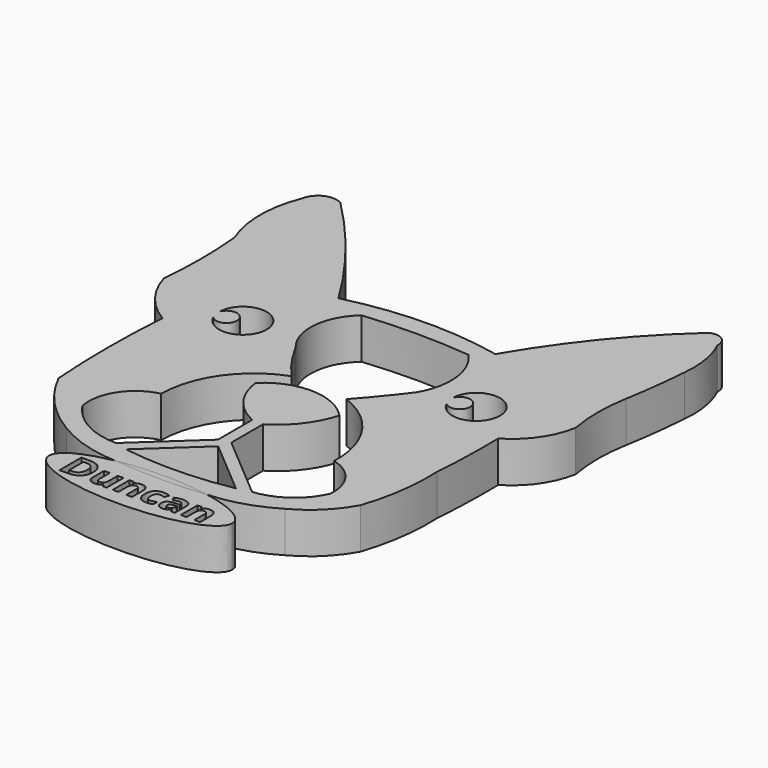
from build123d import *

# Parameters (mm, degrees)
F1_DEPTH     = 10.16
F3_DEPTH     = 10.16
F4_TEXT_SIZE = 9.525
F5_DEPTH     = 5.08


# Not quite as in the source:
# - Text() gives the source's letters only with a copy of the font that has no kerning and outlines rounded to 1/6400 em; it was checked with that copy


with BuildPart() as f1:
    # F0 (on Top) → F1 (new body)
    with BuildSketch(Plane.XY):
        with BuildLine():
            ThreePointArc((46.1094070068, 56.9951225018), (31.5697762687, 41.6882489051), (19.5588854926, 24.326228744))
            ThreePointArc((19.5588854926, 24.326228744), (0.314052465, 26.1919087289), (-18.8508713849, 23.6326014211))
            ThreePointArc((-18.8508713849, 23.6326014211), (-30.3038455944, 40.1584186689), (-43.631359511, 55.2133390192))
            ThreePointArc((-43.631359511, 55.2133390192), (-47.9052299325, 55.4144352292), (-50.5344942393, 52.0390275101))
            ThreePointArc((-50.5344942393, 52.0390275101), (-52.5889945931, 41.507319069), (-50.5344942393, 30.9756106278))
            ThreePointArc((-50.5344942393, 30.9756106278), (-50.0022432343, 20.0013943099), (-50.5344942393, 9.027177992))
            ThreePointArc((-50.5344942393, 9.027177992), (-46.6515086932, 1.4227909007), (-40.2682915589, -4.2480837056))
            ThreePointArc((-40.2682915589, -4.2480837056), (-40.8547601658, -20.3554004232), (-40.2682915589, -36.4627171408))
            ThreePointArc((-40.2682915589, -36.4627171408), (-34.2718067866, -45.2149913023), (-26.0122194997, -51.873771256))
            ThreePointArc((-26.0122194997, -51.873771256), (-17.357949606, -55.5954424929), (-8.0055780709, -56.7269772291))
            ThreePointArc((-8.0055780709, -56.7269772291), (2.0272497606, -57.2919090527), (12.0600775921, -56.7269772291))
            ThreePointArc((12.0600775921, -56.7269772291), (20.508147746, -55.3535059037), (28.3278510388, -51.873771256))
            ThreePointArc((28.3278510388, -51.873771256), (34.3097212842, -47.5040793408), (38.7777723627, -41.5953147808))
            ThreePointArc((38.7777723627, -41.5953147808), (41.1294910578, -31.6374415841), (41.6098287935, -21.4169183548))
            ThreePointArc((41.6098287935, -21.4169183548), (42.1015341125, -12.2192619456), (42.140844077, -3.008555552))
            ThreePointArc((42.140844077, -3.008555552), (48.0273294619, 2.4681230132), (51.0655057607, 9.9121946861))
            ThreePointArc((51.0655057607, 9.9121946861), (50.3560378531, 17.7003484599), (51.0655057607, 25.4885022337))
            ThreePointArc((51.0655057607, 25.4885022337), (52.2263654565, 33.3420013206), (53.0125417352, 41.2418095461))
            ThreePointArc((53.0125417352, 41.2418095461), (52.845884491, 47.8496203591), (50.8885031743, 54.163066071))
            ThreePointArc((50.8885031743, 54.163066071), (49.3865522707, 57.0769148227), (46.1094070068, 56.9951225018))
        make_face()
        with BuildLine():
            ThreePointArc((15.4883818231, -51.1322079441), (2.0678259512, -52.5075336734), (-11.3966716049, -51.6648318688))
            Line((-11.3966716049, -51.6648318688), (1.7883915697, -39.488322453))
            Line((1.7883915697, -39.488322453), (15.4883818231, -51.1322079441))
        make_face(mode=Mode.SUBTRACT)
        with BuildLine():
            ThreePointArc((-12.4149279114, 2.3010451446), (-15.4278442882, 11.8913796265), (-10.8365679733, 20.8341064124))
            ThreePointArc((-10.8365679733, 20.8341064124), (2.4456944574, 21.4907081036), (15.7279568882, 20.8341064124))
            ThreePointArc((15.7279568882, 20.8341064124), (19.7318579177, 11.8860146566), (17.6756650818, 2.3010451446))
            ThreePointArc((17.6756650818, 2.3010451446), (13.360593972, -3.1877374955), (8.8254924978, -8.4961674112))
            ThreePointArc((8.8254924978, -8.4961674112), (19.5314628636, -17.0524210882), (23.1627734759, -30.2675965201))
            ThreePointArc((23.1627734759, -30.2675965201), (29.2997635514, -34.3887895852), (31.1579465623, -41.5437903095))
            ThreePointArc((31.1579465623, -41.5437903095), (26.1919577218, -47.5856552976), (18.8729660916, -50.3420187016))
            Line((18.8729660916, -50.3420187016), (2.794, -36.6761958417))
            Line((2.794, -36.6761958417), (2.794, -26.8115718085))
            ThreePointArc((2.794, -26.8115718085), (8.5855432858, -21.6418194361), (12.0600775921, -14.6994909665))
            ThreePointArc((12.0600775921, -14.6994909665), (1.5615765351, -9.9341013391), (-9.1689196, -14.1511993271))
            ThreePointArc((-9.1689196, -14.1511993271), (-6.2474120303, -21.6344377584), (0, -26.684577046))
            Line((0, -26.684577046), (0, -37.3367219625))
            Line((0, -37.3367219625), (-14.5780167548, -50.7996349518))
            ThreePointArc((-14.5780167548, -50.7996349518), (-23.0306780409, -48.6039650917), (-29.4234489907, -42.654097149))
            ThreePointArc((-29.4234489907, -42.654097149), (-27.7824057255, -34.1107406098), (-20.6442102458, -29.1380020033))
            ThreePointArc((-20.6442102458, -29.1380020033), (-16.4424596943, -16.0090862438), (-5.5117917722, -7.6100603781))
            ThreePointArc((-5.5117917722, -7.6100603781), (-9.2731829133, -2.8703009848), (-12.4149279114, 2.3010451446))
        make_face(mode=Mode.SUBTRACT)
        with BuildLine():
            ThreePointArc((-33.3510132501, 4.8376011459), (-21.635570234, 5.9158243628), (-32.7913214432, 2.1790630207))
            ThreePointArc((-32.7913214432, 2.1790630207), (-28.3838828542, 4.4951280605), (-33.3510132501, 4.8376011459))
        make_face(mode=Mode.SUBTRACT)
        with BuildLine():
            ThreePointArc((24.5965443862, 4.8376011459), (36.3119874023, 5.9158243628), (25.1562361931, 2.1790630207))
            ThreePointArc((25.1562361931, 2.1790630207), (29.5636747821, 4.4951280605), (24.5965443862, 4.8376011459))
        make_face(mode=Mode.SUBTRACT)
    extrude(amount=F1_DEPTH)

    # F2 (on Top) → F3 (join)
    with BuildSketch(Plane.XY):
        with BuildLine():
            add(Edge.make_bspline(
                [(24.1046699662, -63.0293563008), (24.1046699662, -50.3192401212), (-10.018295048, -56.674298211), (-44.1412600622, -63.0293563008), (-10.018295048, -69.3844143907), (24.1046699662, -75.7394724805), (24.1046699662, -63.0293563008)],
                knots=[0, 0, 0, 2.0943951024, 2.0943951024, 4.1887902048, 4.1887902048, 6.2831853072, 6.2831853072, 6.2831853072], degree=2, weights=[1, 0.5, 1, 0.5, 1, 0.5, 1]))
        make_face()
    extrude(amount=F3_DEPTH)

    # F4 (on face) → F5 (cut)
    with BuildSketch(Plane.XY.offset(10.16)):
        with Locations((-16.835979236, -66.5575452986)):
            Text('Duncan', F4_TEXT_SIZE, font='Open Sans', font_style=FontStyle.BOLD, text_align=(TextAlign.LEFT, TextAlign.BOTTOM))
    extrude(amount=-F5_DEPTH, mode=Mode.SUBTRACT)


solid = f1.part
